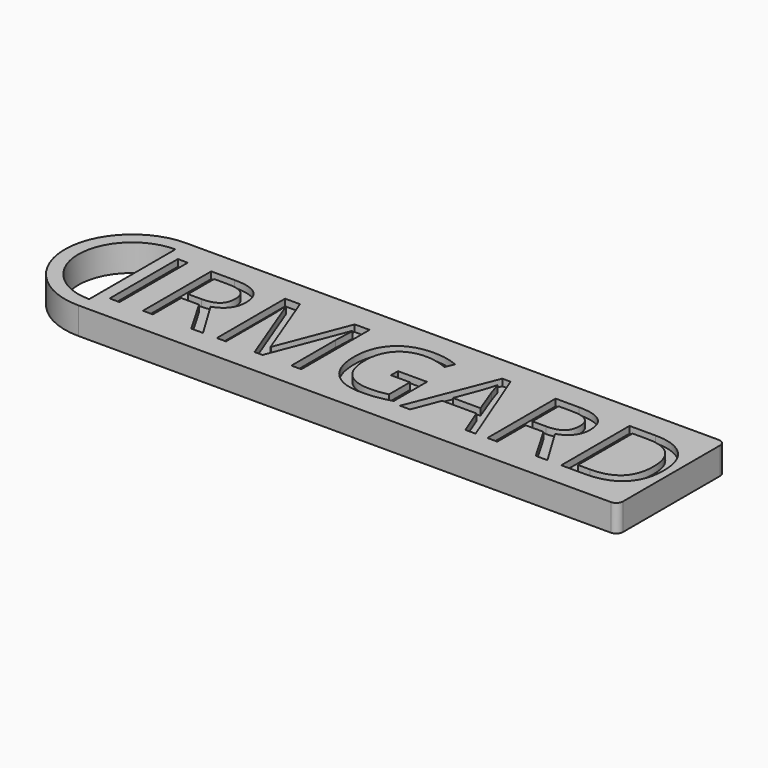
from build123d import *

# Parameters (mm, degrees)
F4_DEPTH     = 2
F1_R         = 0.5
F2_TEXT_SIZE = 8.8664149898
F3_DEPTH     = 0.5


# Not quite as in the source:
# - Text() gives the source's letters only with a copy of the font that has no kerning and outlines rounded to 1/6400 em; it was checked with that copy


with BuildPart() as f4:
    # F0 (on Top) → F4 (new body)
    with BuildSketch(Plane.XY):
        Polygon((34.7291392038, 3.2207785361), (-5.2708607962, 3.2207785361), (-5.2708607962, 2.2207785361), (-5.2708607962, -5.7792214639), (-5.2708607962, -6.7792214639), (34.7291392038, -6.7792214639), align=None)
        with BuildLine():
            Line((-5.2708607962, 2.2207785361), (-5.2708607962, 3.2207785361))
            ThreePointArc((-5.2708607962, 3.2207785361), (-10.2708607962, -1.7792214639), (-5.2708607962, -6.7792214639))
            Line((-5.2708607962, -6.7792214639), (-5.2708607962, -5.7792214639))
            ThreePointArc((-5.2708607962, -5.7792214639), (-9.2708607962, -1.7792214639), (-5.2708607962, 2.2207785361))
        make_face()
    extrude(amount=F4_DEPTH)

    # F1
    f1_edges = [f4.edges().sort_by_distance(p)[0] for p in [
        (34.729139, -6.779221, 1),
        (34.729139, 3.220779, 1),
    ]]
    fillet(f1_edges, radius=F1_R)

    # F2 (on face) → F3 (cut)
    with BuildSketch(Plane.XY.offset(2)):
        with Locations((-5.2708607962, -4.9711308603)):
            Text('IRMGARD', F2_TEXT_SIZE, font='Open Sans', text_align=(TextAlign.LEFT, TextAlign.BOTTOM))
    extrude(amount=-F3_DEPTH, mode=Mode.SUBTRACT)


solid = f4.part
